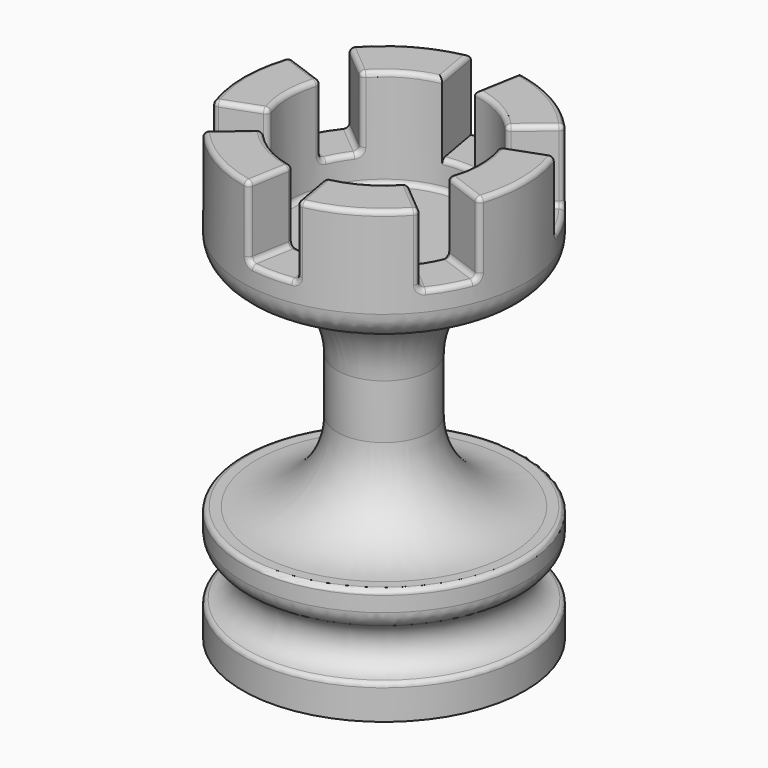
from build123d import *

# Parameters (mm, degrees)
F2_R     = 20
F3_DEPTH = 21
F5_DEPTH = 15
F6_R     = 17
F7_R     = 6
F8_F1_R  = 1
F8_F2_R  = 1
F9_R     = 1
F10_R    = 4


with BuildPart() as f1:
    # F0 (on Front) → F1 (revolve)
    with BuildSketch(Plane.XZ):
        with BuildLine():
            Line((29.8611142606, 24.5238091864), (9.8611142606, 24.5238091864))
            Line((9.8611142606, 24.5238091864), (9.8611142606, 70))
            Line((9.8611142606, 70), (29.8611142606, 70))
            Line((29.8611142606, 70), (29.8611142606, 95))
            Line((29.8611142606, 95), (0, 95))
            Line((0, 95), (0, 0))
            Line((0, 0), (29.8611142606, 0))
            Line((29.8611142606, 0), (29.8611142606, 7.2619045932))
            ThreePointArc((29.8611142606, 7.2619045932), (24.8611142606, 12.2619045932), (29.8611142606, 17.2619045932))
            Line((29.8611142606, 17.2619045932), (29.8611142606, 24.5238091864))
        make_face()
    revolve(axis=Axis((0, 0, 47.5), (0, 0, -1)))

    # F2 (on face) → F3 (cut)
    with BuildSketch(Plane.XY.offset(95)):
        Circle(F2_R)
    extrude(amount=-F3_DEPTH, mode=Mode.SUBTRACT)

    # F4 (on face) → F5 (cut)
    with BuildSketch(Plane.XY.offset(95)):
        with BuildLine():
            ThreePointArc((-3.4729635533, 19.6961550602), (0, 20), (3.4729635533, 19.6961550602))
            Line((3.4729635533, 19.6961550602), (5.20944533, 29.5442325904))
            ThreePointArc((5.20944533, 29.5442325904), (0, 30), (-5.20944533, 29.5442325904))
            Line((-5.20944533, 29.5442325904), (-3.4729635533, 19.6961550602))
        make_face()
        with BuildLine():
            Line((-28.1907786236, 10.2606042998), (-18.7938524157, 6.8404028665))
            ThreePointArc((-18.7938524157, 6.8404028665), (-17.3205080757, 10), (-15.3208888624, 12.8557521937))
            Line((-15.3208888624, 12.8557521937), (-22.9813332936, 19.2836282906))
            ThreePointArc((-22.9813332936, 19.2836282906), (-25.9807621135, 15), (-28.1907786236, 10.2606042998))
        make_face()
        with BuildLine():
            Line((-22.9813332936, -19.2836282906), (-15.3208888624, -12.8557521937))
            ThreePointArc((-15.3208888624, -12.8557521937), (-17.3205080757, -10), (-18.7938524157, -6.8404028665))
            Line((-18.7938524157, -6.8404028665), (-28.1907786236, -10.2606042998))
            ThreePointArc((-28.1907786236, -10.2606042998), (-25.9807621135, -15), (-22.9813332936, -19.2836282906))
        make_face()
        with BuildLine():
            Line((5.20944533, -29.5442325904), (3.4729635533, -19.6961550602))
            ThreePointArc((3.4729635533, -19.6961550602), (0, -20), (-3.4729635533, -19.6961550602))
            Line((-3.4729635533, -19.6961550602), (-5.20944533, -29.5442325904))
            ThreePointArc((-5.20944533, -29.5442325904), (0, -30), (5.20944533, -29.5442325904))
        make_face()
        with BuildLine():
            Line((28.1907786236, -10.2606042998), (18.7938524157, -6.8404028665))
            ThreePointArc((18.7938524157, -6.8404028665), (17.3205080757, -10), (15.3208888624, -12.8557521937))
            Line((15.3208888624, -12.8557521937), (22.9813332936, -19.2836282906))
            ThreePointArc((22.9813332936, -19.2836282906), (25.9807621135, -15), (28.1907786236, -10.2606042998))
        make_face()
        with BuildLine():
            Line((22.9813332936, 19.2836282906), (15.3208888624, 12.8557521937))
            ThreePointArc((15.3208888624, 12.8557521937), (17.3205080757, 10), (18.7938524157, 6.8404028665))
            Line((18.7938524157, 6.8404028665), (28.1907786236, 10.2606042998))
            ThreePointArc((28.1907786236, 10.2606042998), (25.9807621135, 15), (22.9813332936, 19.2836282906))
        make_face()
    extrude(amount=-F5_DEPTH, mode=Mode.SUBTRACT)

    # F6
    f6_edges = [f1.edges().sort_by_distance(p)[0] for p in [
        (-9.861114, 0, 24.523809),
        (-9.861114, 0, 70),
        (9.861114, 0, 47.261905),
    ]]
    fillet(f6_edges, radius=F6_R)

    # F7
    f7_edges = [f1.edges().sort_by_distance(p)[0] for p in [
        (-29.861114, 0, 70),
    ]]
    fillet(f7_edges, radius=F7_R)

    # F8: fillet of radius 1 on 49 edges, made by hand

    # F8_f1
    f8_f1_edges = [f1.edges().sort_by_distance(p)[0] for p in [
        (-20, 0, 74),
        (-23.4270605674, 8.5267527229, 80),
        (-19.0979147535, 16.0250532259, 80),
        (19.0979147535, -16.0250532259, 80),
        (23.4270605674, -8.5267527229, 80),
        (-4.3291458139, -24.5518059488, 80),
        (4.3291458139, -24.5518059488, 80),
        (-19.0979147535, -16.0250532259, 80),
        (-23.4270605674, -8.5267527229, 80),
        (23.4270605674, 8.5267527229, 80),
        (19.0979147535, 16.0250532259, 80),
    ]]
    fillet(f8_f1_edges, radius=F8_F1_R)

    # F8_f2
    f8_f2_edges = [f1.edges().sort_by_distance(p)[0] for p in [
        (-29.8611142606, 0, 24.5238091864),
        (19.0979147535, -16.0250532259, 95),
        (10, -17.3205080757, 95),
        (4.3291458139, -24.5518059488, 95),
        (14.9305571303, -25.860483535, 95),
        (29.4074568374, 5.1853280745, 95),
        (23.4270605674, 8.5267527229, 95),
        (19.6961550602, 3.4729635533, 95),
        (19.6961550602, -3.4729635533, 95),
        (23.4270605674, -8.5267527229, 95),
        (29.4074568374, -5.1853280745, 95),
        (14.9305571303, 25.860483535, 95),
        (4.3291458139, 24.5518059488, 95),
        (10, 17.3205080757, 95),
        (19.0979147535, 16.0250532259, 95),
        (-14.9305571303, 25.860483535, 95),
        (-19.0979147535, 16.0250532259, 95),
        (-10, 17.3205080757, 95),
        (-4.3291458139, 24.5518059488, 95),
        (-23.4270605674, -8.5267527229, 95),
        (-20, 0, 95),
        (-23.4270605674, 8.5267527229, 95),
        (-29.8611142606, 0, 95),
        (-4.3291458139, -24.5518059488, 95),
        (-10, -17.3205080757, 95),
        (-19.0979147535, -16.0250532259, 95),
        (-14.9305571303, -25.860483535, 95),
        (-17.3205080757, 10, 80),
        (-25.860483535, 14.9305571303, 80),
        (0, 20, 80),
        (25.860483535, 14.9305571303, 80),
        (25.860483535, -14.9305571303, 80),
        (17.3205080757, -10, 80),
        (0, -29.8611142606, 80),
        (0, -20, 80),
        (-17.3205080757, -10, 80),
        (-25.860483535, -14.9305571303, 80),
        (17.3205080757, 10, 80),
        (15.4855125986, 12.6569703952, 80.3294963101),
        (18.7039671591, 7.0824863232, 80.3293493917),
        (-27.9709870931, -10.4551435165, 80.3296220208),
        (-23.0399970557, -18.9959122067, 80.3294765648),
        (-15.4855966574, -12.6568675497, 80.3293493917),
        (-18.7040141964, -7.0823621034, 80.3294963101),
        (3.2183793993, -19.7393524224, 80.3293593562),
        (-3.2185015979, -19.7393324986, 80.3294963101),
        (-4.931073661, -29.4511571498, 80.3296220208),
        (4.9309528338, -29.4511773797, 80.329486456),
        (18.7039703517, -7.0824778924, 80.3293593562),
        (15.4855125986, -12.6569703952, 80.3294963101),
        (23.039913432, -18.9960136333, 80.3296220208),
        (27.9709441991, -10.4552582709, 80.329486456),
        (27.9709410669, 10.45526665, 80.3294765648),
        (23.039913432, 18.9960136333, 80.3296220208),
        (-23.0399913653, 18.9959191088, 80.329486456),
        (-27.9709870931, 10.4551435165, 80.3296220208),
        (-18.7040141964, 7.0823621034, 80.3294963101),
        (-15.4855909524, 12.65687453, 80.3293593562),
    ]]
    fillet(f8_f2_edges, radius=F8_F2_R)

    # F9
    f9_edges = [f1.edges().sort_by_distance(p)[0] for p in [
        (-29.861114, 0, 7.261905),
    ]]
    fillet(f9_edges, radius=F9_R)

    # F10
    f10_edges = [f1.edges().sort_by_distance(p)[0] for p in [
        (-29.861114, 0, 17.261905),
    ]]
    fillet(f10_edges, radius=F10_R)


solid = f1.part
